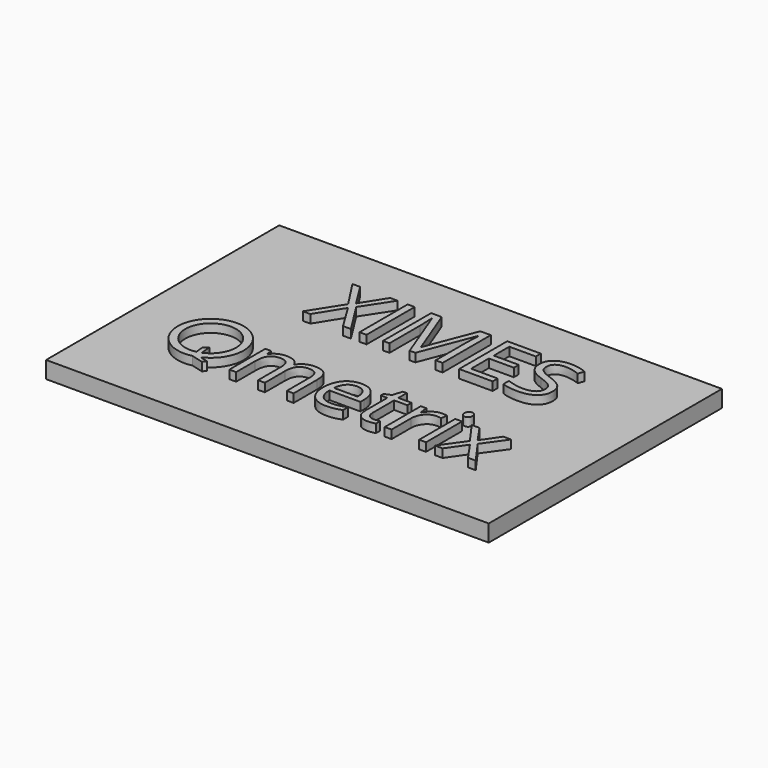
from build123d import *

# Parameters (mm, degrees)
F0_W         = 261.7531362921
F0_H         = 172.3503917456
F0_W_2       = 4.0420560748
F0_H_2       = 26.6744548287
F0_W_3       = 4.1355140187
F0_H_3       = 35.5841121495
F1_DEPTH     = 10
F0_TEXT_SIZE = 49.8442367601
F2_DEPTH     = 15


# Not quite as in the source:
# - Text() gives the source's letters only with a copy of the font that has no kerning and outlines rounded to 1/6400 em; it was checked with that copy


with BuildPart() as f1:
    # F0 (on Top) → F1 (new body)
    with BuildSketch(Plane.XY):
        with Locations((29.5447735116, 5.9954747558)):
            Rectangle(F0_W, F0_H)
        with BuildLine():
            ThreePointArc((-45.0583331062, -42.3228889704), (-55.8059475031, -4.8705779818), (-41.2665927015, -41.0201834508))
            Line((-41.2665927015, -41.0201834508), (-36.3650284708, -42.3228889704))
            Line((-36.3650284708, -42.3228889704), (-37.9992168005, -44.1990144973))
            Line((-37.9992168005, -44.1990144973), (-45.0583331062, -42.3228889704))
        make_face(mode=Mode.SUBTRACT)
        with BuildLine():
            Line((14.8038502761, -42.3830400759), (10.7695823634, -42.3830400759))
            Line((10.7695823634, -42.3830400759), (10.7695823634, -25.0310151538))
            add(Edge.make_bspline(
                [(10.7695823634, -25.0310151538), (10.7695823634, -21.8378687364), (9.4066540145, -20.2451896086)],
                knots=[0, 0, 0, 1, 1, 1], degree=2))
            add(Edge.make_bspline(
                [(9.4066540145, -20.2451896086), (8.0437256656, -18.6525104809), (5.1698938899, -18.6525104809)],
                knots=[0, 0, 0, 1, 1, 1], degree=2))
            add(Edge.make_bspline(
                [(5.1698938899, -18.6525104809), (1.4004234849, -18.6525104809), (-0.4025360167, -20.8176195152)],
                knots=[0, 0, 0, 1, 1, 1], degree=2))
            add(Edge.make_bspline(
                [(-0.4025360167, -20.8176195152), (-2.2054955182, -22.9827285495), (-2.2054955182, -27.4842861819)],
                knots=[0, 0, 0, 1, 1, 1], degree=2))
            Line((-2.2054955182, -27.4842861819), (-2.2054955182, -42.3830400759))
            Line((-2.2054955182, -42.3830400759), (-6.247551593, -42.3830400759))
            Line((-6.247551593, -42.3830400759), (-6.247551593, -25.0310151538))
            add(Edge.make_bspline(
                [(-6.247551593, -25.0310151538), (-6.247551593, -21.8378687364), (-7.6104799419, -20.2451896086)],
                knots=[0, 0, 0, 1, 1, 1], degree=2))
            add(Edge.make_bspline(
                [(-7.6104799419, -20.2451896086), (-8.9734082908, -18.6525104809), (-11.8706045525, -18.6525104809)],
                knots=[0, 0, 0, 1, 1, 1], degree=2))
            add(Edge.make_bspline(
                [(-11.8706045525, -18.6525104809), (-15.6634394435, -18.6525104809), (-17.4274581351, -20.9266537831)],
                knots=[0, 0, 0, 1, 1, 1], degree=2))
            add(Edge.make_bspline(
                [(-17.4274581351, -20.9266537831), (-19.1914768267, -23.2007970853), (-19.1914768267, -28.3877129731)],
                knots=[0, 0, 0, 1, 1, 1], degree=2))
            Line((-19.1914768267, -28.3877129731), (-19.1914768267, -42.3830400759))
            Line((-19.1914768267, -42.3830400759), (-23.2335329014, -42.3830400759))
            Line((-23.2335329014, -42.3830400759), (-23.2335329014, -15.7085852473))
            Line((-23.2335329014, -15.7085852473), (-19.9469285401, -15.7085852473))
            Line((-19.9469285401, -15.7085852473), (-19.2927229326, -19.3612332224))
            Line((-19.2927229326, -19.3612332224), (-19.0980188827, -19.3612332224))
            add(Edge.make_bspline(
                [(-19.0980188827, -19.3612332224), (-17.9531590696, -17.4141927239), (-15.8698257363, -16.3160618828)],
                knots=[0, 0, 0, 1, 1, 1], degree=2))
            add(Edge.make_bspline(
                [(-15.8698257363, -16.3160618828), (-13.786492403, -15.2179310417), (-11.208610783, -15.2179310417)],
                knots=[0, 0, 0, 1, 1, 1], degree=2))
            add(Edge.make_bspline(
                [(-11.208610783, -15.2179310417), (-4.954716702, -15.2179310417), (-3.0310406896, -19.750641322)],
                knots=[0, 0, 0, 1, 1, 1], degree=2))
            Line((-3.0310406896, -19.750641322), (-2.8363366397, -19.750641322))
            add(Edge.make_bspline(
                [(-2.8363366397, -19.750641322), (-1.6447478547, -17.6556257457), (0.6177132045, -16.4367783937)],
                knots=[0, 0, 0, 1, 1, 1], degree=2))
            add(Edge.make_bspline(
                [(0.6177132045, -16.4367783937), (2.8801742637, -15.2179310417), (5.7773705254, -15.2179310417)],
                knots=[0, 0, 0, 1, 1, 1], degree=2))
            add(Edge.make_bspline(
                [(5.7773705254, -15.2179310417), (10.3022926437, -15.2179310417), (12.5530714599, -17.5426973968)],
                knots=[0, 0, 0, 1, 1, 1], degree=2))
            add(Edge.make_bspline(
                [(12.5530714599, -17.5426973968), (14.8038502761, -19.8674637519), (14.8038502761, -24.9842861819)],
                knots=[0, 0, 0, 1, 1, 1], degree=2))
            Line((14.8038502761, -24.9842861819), (14.8038502761, -42.3830400759))
        make_face(mode=Mode.SUBTRACT)
        with BuildLine():
            add(Edge.make_bspline(
                [(39.0094577528, -42.4687098579), (37.1013580643, -42.8736942815), (34.3988658525, -42.8736942815)],
                knots=[0, 0, 0, 1, 1, 1], degree=2))
            add(Edge.make_bspline(
                [(34.3988658525, -42.8736942815), (28.4876508992, -42.8736942815), (25.0647537029, -39.2677752784)],
                knots=[0, 0, 0, 1, 1, 1], degree=2))
            add(Edge.make_bspline(
                [(25.0647537029, -39.2677752784), (21.6418565067, -35.6618562753), (21.6418565067, -29.2677752784)],
                knots=[0, 0, 0, 1, 1, 1], degree=2))
            add(Edge.make_bspline(
                [(21.6418565067, -29.2677752784), (21.6418565067, -22.8113889856), (24.8194266001, -19.0146600136)],
                knots=[0, 0, 0, 1, 1, 1], degree=2))
            add(Edge.make_bspline(
                [(24.8194266001, -19.0146600136), (27.9969966936, -15.2179310417), (33.3552521453, -15.2179310417)],
                knots=[0, 0, 0, 1, 1, 1], degree=2))
            add(Edge.make_bspline(
                [(33.3552521453, -15.2179310417), (38.3630403073, -15.2179310417), (41.283601055, -18.516217646)],
                knots=[0, 0, 0, 1, 1, 1], degree=2))
            add(Edge.make_bspline(
                [(41.283601055, -18.516217646), (44.2041618026, -21.8145042504), (44.2041618026, -27.2194886741)],
                knots=[0, 0, 0, 1, 1, 1], degree=2))
            Line((44.2041618026, -27.2194886741), (44.2041618026, -29.774005808))
            Line((44.2041618026, -29.774005808), (25.8318876593, -29.774005808))
            add(Edge.make_bspline(
                [(25.8318876593, -29.774005808), (25.9564982512, -34.4702674903), (28.2072770674, -36.9040681133)],
                knots=[0, 0, 0, 1, 1, 1], degree=2))
            add(Edge.make_bspline(
                [(28.2072770674, -36.9040681133), (30.4580558836, -39.3378687364), (34.5468409304, -39.3378687364)],
                knots=[0, 0, 0, 1, 1, 1], degree=2))
            add(Edge.make_bspline(
                [(34.5468409304, -39.3378687364), (38.8536945129, -39.3378687364), (43.0593019895, -37.5388033158)],
                knots=[0, 0, 0, 1, 1, 1], degree=2))
            Line((43.0593019895, -37.5388033158), (43.0593019895, -41.1447223189))
            add(Edge.make_bspline(
                [(43.0593019895, -41.1447223189), (40.9175574413, -42.0637254342), (39.0094577528, -42.4687098579)],
                knots=[0, 0, 0, 1, 1, 1], degree=2))
        make_face(mode=Mode.SUBTRACT)
        with BuildLine():
            add(Edge.make_bspline(
                [(56.5717630487, -38.2436319762), (57.7166228618, -39.5325727862), (59.7103923322, -39.5325727862)],
                knots=[0, 0, 0, 1, 1, 1], degree=2))
            add(Edge.make_bspline(
                [(59.7103923322, -39.5325727862), (60.7851586874, -39.5325727862), (61.7820434226, -39.3768095463)],
                knots=[0, 0, 0, 1, 1, 1], degree=2))
            add(Edge.make_bspline(
                [(61.7820434226, -39.3768095463), (62.7789281578, -39.2210463065), (63.3630403073, -39.0497067426)],
                knots=[0, 0, 0, 1, 1, 1], degree=2))
            Line((63.3630403073, -39.0497067426), (63.3630403073, -42.1416070541))
            add(Edge.make_bspline(
                [(63.3630403073, -42.1416070541), (62.7088346998, -42.4531335339), (61.4315761328, -42.6634139077)],
                knots=[0, 0, 0, 1, 1, 1], degree=2))
            add(Edge.make_bspline(
                [(61.4315761328, -42.6634139077), (60.1543175659, -42.8736942815), (59.1262801827, -42.8736942815)],
                knots=[0, 0, 0, 1, 1, 1], degree=2))
            add(Edge.make_bspline(
                [(59.1262801827, -42.8736942815), (51.3926353229, -42.8736942815), (51.3926353229, -34.7194886741)],
                knots=[0, 0, 0, 1, 1, 1], degree=2))
            Line((51.3926353229, -34.7194886741), (51.3926353229, -18.8472145308))
            Line((51.3926353229, -18.8472145308), (47.5686477839, -18.8472145308))
            Line((47.5686477839, -18.8472145308), (47.5686477839, -16.9001740323))
            Line((47.5686477839, -16.9001740323), (51.3926353229, -15.2179310417))
            Line((51.3926353229, -15.2179310417), (53.0904546375, -9.5247846242))
            Line((53.0904546375, -9.5247846242), (55.4269032356, -9.5247846242))
            Line((55.4269032356, -9.5247846242), (55.4269032356, -15.7085852473))
            Line((55.4269032356, -15.7085852473), (63.1683362575, -15.7085852473))
            Line((63.1683362575, -15.7085852473), (63.1683362575, -18.8472145308))
            Line((63.1683362575, -18.8472145308), (55.4269032356, -18.8472145308))
            Line((55.4269032356, -18.8472145308), (55.4269032356, -34.5481491102))
            add(Edge.make_bspline(
                [(55.4269032356, -34.5481491102), (55.4269032356, -36.9546911663), (56.5717630487, -38.2436319762)],
                knots=[0, 0, 0, 1, 1, 1], degree=2))
        make_face(mode=Mode.SUBTRACT)
        with BuildLine():
            add(Edge.make_bspline(
                [(76.260236569, -16.6314824435), (78.3552521453, -15.2179310417), (80.8630403073, -15.2179310417)],
                knots=[0, 0, 0, 1, 1, 1], degree=2))
            add(Edge.make_bspline(
                [(80.8630403073, -15.2179310417), (82.6387412419, -15.2179310417), (84.0483985628, -15.5138811974)],
                knots=[0, 0, 0, 1, 1, 1], degree=2))
            Line((84.0483985628, -15.5138811974), (83.4876508992, -19.2599871164))
            add(Edge.make_bspline(
                [(83.4876508992, -19.2599871164), (81.8365605565, -18.8939435027), (80.5670901515, -18.8939435027)],
                knots=[0, 0, 0, 1, 1, 1], degree=2))
            add(Edge.make_bspline(
                [(80.5670901515, -18.8939435027), (77.3272147621, -18.8939435027), (75.029706974, -21.5224481756)],
                knots=[0, 0, 0, 1, 1, 1], degree=2))
            add(Edge.make_bspline(
                [(75.029706974, -21.5224481756), (72.7321991858, -24.1509528485), (72.7321991858, -28.0683983314)],
                knots=[0, 0, 0, 1, 1, 1], degree=2))
            Line((72.7321991858, -28.0683983314), (72.7321991858, -42.3830400759))
            Line((72.7321991858, -42.3830400759), (68.690143111, -42.3830400759))
            Line((68.690143111, -42.3830400759), (68.690143111, -15.7085852473))
            Line((68.690143111, -15.7085852473), (72.0234764444, -15.7085852473))
            Line((72.0234764444, -15.7085852473), (72.490766164, -20.6462799513))
            Line((72.490766164, -20.6462799513), (72.6854702138, -20.6462799513))
            add(Edge.make_bspline(
                [(72.6854702138, -20.6462799513), (74.1652209927, -18.0450338454), (76.260236569, -16.6314824435)],
                knots=[0, 0, 0, 1, 1, 1], degree=2))
        make_face(mode=Mode.SUBTRACT)
        with Locations((91.0616384381, -29.0458126616)):
            Rectangle(F0_W_2, F0_H_2, mode=Mode.SUBTRACT)
        with BuildLine():
            add(Edge.make_bspline(
                [(89.3793954475, -10.5138811974), (88.697931273, -9.844099266), (88.697931273, -8.4811709171)],
                knots=[0, 0, 0, 1, 1, 1], degree=2))
            add(Edge.make_bspline(
                [(88.697931273, -8.4811709171), (88.697931273, -7.0948780822), (89.3793954475, -6.4484606367)],
                knots=[0, 0, 0, 1, 1, 1], degree=2))
            add(Edge.make_bspline(
                [(89.3793954475, -6.4484606367), (90.0608596219, -5.8020431912), (91.0888970051, -5.8020431912)],
                knots=[0, 0, 0, 1, 1, 1], degree=2))
            add(Edge.make_bspline(
                [(91.0888970051, -5.8020431912), (92.0624172543, -5.8020431912), (92.7672459148, -6.4601428797)],
                knots=[0, 0, 0, 1, 1, 1], degree=2))
            add(Edge.make_bspline(
                [(92.7672459148, -6.4601428797), (93.4720745752, -7.1182425681), (93.4720745752, -8.4811709171)],
                knots=[0, 0, 0, 1, 1, 1], degree=2))
            add(Edge.make_bspline(
                [(93.4720745752, -8.4811709171), (93.4720745752, -9.844099266), (92.7672459148, -10.5138811974)],
                knots=[0, 0, 0, 1, 1, 1], degree=2))
            add(Edge.make_bspline(
                [(92.7672459148, -10.5138811974), (92.0624172543, -11.1836631289), (91.0888970051, -11.1836631289)],
                knots=[0, 0, 0, 1, 1, 1], degree=2))
            add(Edge.make_bspline(
                [(91.0888970051, -11.1836631289), (90.0608596219, -11.1836631289), (89.3793954475, -10.5138811974)],
                knots=[0, 0, 0, 1, 1, 1], degree=2))
        make_face(mode=Mode.SUBTRACT)
        Polygon((98.3163113353, -42.3830400759), (108.0748783135, -28.7303921009), (98.799177379, -15.7085852473), (103.4019811173, -15.7085852473), (110.4346913976, -25.9266537831), (117.444037192, -15.7085852473), (122.0001119584, -15.7085852473), (112.7244110238, -28.7303921009), (122.482978002, -42.3830400759), (117.9113269117, -42.3830400759), (110.4346913976, -31.5730712286), (102.8879624257, -42.3830400759), align=None, mode=Mode.SUBTRACT)
        Polygon((-16.6011314449, 43.1183571619), (-4.7241844044, 24.3800394049), (-9.4204460866, 24.3800394049), (-18.984309015, 40.0264568504), (-28.7195115072, 24.3800394049), (-33.1042467097, 24.3800394049), (-21.2740286411, 42.978170246), (-32.3020660243, 59.9641515544), (-27.722626772, 59.9641515544), (-18.8908510711, 45.8675783457), (-9.9811937502, 59.9641515544), (-5.5808822237, 59.9641515544), align=None, mode=Mode.SUBTRACT)
        with Locations((2.4292423869, 42.1720954797)):
            Rectangle(F0_W_3, F0_H_3, mode=Mode.SUBTRACT)
        with BuildLine():
            Line((33.3365632592, 24.3800394049), (30.0032299258, 24.3800394049))
            Line((30.0032299258, 24.3800394049), (17.9315788355, 55.9220954797))
            Line((17.9315788355, 55.9220954797), (17.7368747856, 55.9220954797))
            add(Edge.make_bspline(
                [(17.7368747856, 55.9220954797), (18.0795539134, 52.1759895607), (18.0795539134, 47.0124381588)],
                knots=[0, 0, 0, 1, 1, 1], degree=2))
            Line((18.0795539134, 47.0124381588), (18.0795539134, 24.3800394049))
            Line((18.0795539134, 24.3800394049), (14.2555663744, 24.3800394049))
            Line((14.2555663744, 24.3800394049), (14.2555663744, 59.9641515544))
            Line((14.2555663744, 59.9641515544), (20.4860959694, 59.9641515544))
            Line((20.4860959694, 59.9641515544), (31.7555663744, 30.6105689999))
            Line((31.7555663744, 30.6105689999), (31.9502704243, 30.6105689999))
            Line((31.9502704243, 30.6105689999), (43.3131987732, 59.9641515544))
            Line((43.3131987732, 59.9641515544), (49.4969993962, 59.9641515544))
            Line((49.4969993962, 59.9641515544), (49.4969993962, 24.3800394049))
            Line((49.4969993962, 24.3800394049), (45.3614853775, 24.3800394049))
            Line((45.3614853775, 24.3800394049), (45.3614853775, 47.3083883146))
            add(Edge.make_bspline(
                [(45.3614853775, 47.3083883146), (45.3614853775, 51.2491982834), (45.7041645053, 55.8753665077)],
                knots=[0, 0, 0, 1, 1, 1], degree=2))
            Line((45.7041645053, 55.8753665077), (45.5094604554, 55.8753665077))
            Line((45.5094604554, 55.8753665077), (33.3365632592, 24.3800394049))
        make_face(mode=Mode.SUBTRACT)
        Polygon((79.0920149726, 28.0794163519), (79.0920149726, 24.3800394049), (59.2555663744, 24.3800394049), (59.2555663744, 59.9641515544), (79.0920149726, 59.9641515544), (79.0920149726, 56.2881390934), (63.3910803931, 56.2881390934), (63.3910803931, 44.8239646385), (78.1418592093, 44.8239646385), (78.1418592093, 41.1713166635), (63.3910803931, 41.1713166635), (63.3910803931, 28.0794163519), align=None, mode=Mode.SUBTRACT)
        with BuildLine():
            add(Edge.make_bspline(
                [(104.9487127919, 39.7850238286), (107.0515165302, 37.4953042024), (107.0515165302, 33.8504443893)],
                knots=[0, 0, 0, 1, 1, 1], degree=2))
            add(Edge.make_bspline(
                [(107.0515165302, 33.8504443893), (107.0515165302, 29.1541827071), (103.6441956579, 26.5217839532)],
                knots=[0, 0, 0, 1, 1, 1], degree=2))
            add(Edge.make_bspline(
                [(103.6441956579, 26.5217839532), (100.2368747856, 23.8893851993), (94.3957532903, 23.8893851993)],
                knots=[0, 0, 0, 1, 1, 1], degree=2))
            add(Edge.make_bspline(
                [(94.3957532903, 23.8893851993), (88.0717657514, 23.8893851993), (84.6605507981, 25.524899218)],
                knots=[0, 0, 0, 1, 1, 1], degree=2))
            Line((84.6605507981, 25.524899218), (84.6605507981, 29.5124381588))
            add(Edge.make_bspline(
                [(84.6605507981, 29.5124381588), (86.8568124803, 28.5934350435), (89.4346941003, 28.056051866)],
                knots=[0, 0, 0, 1, 1, 1], degree=2))
            add(Edge.make_bspline(
                [(89.4346941003, 28.056051866), (92.0125757202, 27.5186686884), (94.5437283682, 27.5186686884)],
                knots=[0, 0, 0, 1, 1, 1], degree=2))
            add(Edge.make_bspline(
                [(94.5437283682, 27.5186686884), (98.6792423869, 27.5186686884), (100.7742579632, 29.0879833301)],
                knots=[0, 0, 0, 1, 1, 1], degree=2))
            add(Edge.make_bspline(
                [(100.7742579632, 29.0879833301), (102.8692735395, 30.6572979719), (102.8692735395, 33.4610362896)],
                knots=[0, 0, 0, 1, 1, 1], degree=2))
            add(Edge.make_bspline(
                [(102.8692735395, 33.4610362896), (102.8692735395, 35.3068306822), (102.1255040691, 36.4867372242)],
                knots=[0, 0, 0, 1, 1, 1], degree=2))
            add(Edge.make_bspline(
                [(102.1255040691, 36.4867372242), (101.3817345987, 37.6666437663), (99.6410803931, 38.6674225825)],
                knots=[0, 0, 0, 1, 1, 1], degree=2))
            add(Edge.make_bspline(
                [(99.6410803931, 38.6674225825), (97.9004261875, 39.6682013987), (94.3490243184, 40.9298836417)],
                knots=[0, 0, 0, 1, 1, 1], degree=2))
            add(Edge.make_bspline(
                [(94.3490243184, 40.9298836417), (89.3879651283, 42.7055845762), (87.257902823, 45.1393851993)],
                knots=[0, 0, 0, 1, 1, 1], degree=2))
            add(Edge.make_bspline(
                [(87.257902823, 45.1393851993), (85.1278405177, 47.5731858223), (85.1278405177, 51.4906313052)],
                knots=[0, 0, 0, 1, 1, 1], degree=2))
            add(Edge.make_bspline(
                [(85.1278405177, 51.4906313052), (85.1278405177, 55.6027808379), (88.2158467483, 58.036581461)],
                knots=[0, 0, 0, 1, 1, 1], degree=2))
            add(Edge.make_bspline(
                [(88.2158467483, 58.036581461), (91.3038529788, 60.470382084), (96.3973109227, 60.470382084)],
                knots=[0, 0, 0, 1, 1, 1], degree=2))
            add(Edge.make_bspline(
                [(96.3973109227, 60.470382084), (101.7010492405, 60.470382084), (106.1558779009, 58.5233415856)],
                knots=[0, 0, 0, 1, 1, 1], degree=2))
            Line((106.1558779009, 58.5233415856), (104.8630430099, 54.9252107445))
            add(Edge.make_bspline(
                [(104.8630430099, 54.9252107445), (100.4549433215, 56.771005137), (96.2960648168, 56.771005137)],
                knots=[0, 0, 0, 1, 1, 1], degree=2))
            add(Edge.make_bspline(
                [(96.2960648168, 56.771005137), (93.0094604554, 56.771005137), (91.1597719819, 55.3613478161)],
                knots=[0, 0, 0, 1, 1, 1], degree=2))
            add(Edge.make_bspline(
                [(91.1597719819, 55.3613478161), (89.3100835084, 53.9516904952), (89.3100835084, 51.4439023333)],
                knots=[0, 0, 0, 1, 1, 1], degree=2))
            add(Edge.make_bspline(
                [(89.3100835084, 51.4439023333), (89.3100835084, 49.5981079407), (89.9915476828, 48.4143073177)],
                knots=[0, 0, 0, 1, 1, 1], degree=2))
            add(Edge.make_bspline(
                [(89.9915476828, 48.4143073177), (90.6730118573, 47.2305066946), (92.292949552, 46.2453042024)],
                knots=[0, 0, 0, 1, 1, 1], degree=2))
            add(Edge.make_bspline(
                [(92.292949552, 46.2453042024), (93.9128872467, 45.2601017102), (97.24622058, 44.0685129252)],
                knots=[0, 0, 0, 1, 1, 1], degree=2))
            add(Edge.make_bspline(
                [(97.24622058, 44.0685129252), (102.8459090536, 42.0747434547), (104.9487127919, 39.7850238286)],
                knots=[0, 0, 0, 1, 1, 1], degree=2))
        make_face(mode=Mode.SUBTRACT)
    extrude(amount=F1_DEPTH)



with BuildPart() as f1b:
    # F0 (on Top) → F1, piece 2 (new body)
    with BuildSketch(Plane.XY):
        with BuildLine():
            ThreePointArc((-43.7490858011, -37.1871398378), (-53.9394303244, -9.0020291393), (-46.276672768, -37.9765995973))
            Line((-46.276672768, -37.9765995973), (-46.6589570613, -33.0732026998))
            Line((-46.6589570613, -33.0732026998), (-44.2494047513, -30.769762951))
            Line((-44.2494047513, -30.769762951), (-43.7490858011, -37.1871398378))
        make_face()
    extrude(amount=F1_DEPTH)


with BuildPart() as f1c:
    # F0 (on Top) → F1, piece 3 (new body)
    with BuildSketch(Plane.XY):
        with BuildLine():
            add(Edge.make_bspline(
                [(38.1722303385, -20.6384917893), (36.4705169428, -18.605781509), (33.3007350114, -18.605781509)],
                knots=[0, 0, 0, 1, 1, 1], degree=2))
            add(Edge.make_bspline(
                [(33.3007350114, -18.605781509), (30.0920122699, -18.605781509), (28.1800185004, -20.6969030043)],
                knots=[0, 0, 0, 1, 1, 1], degree=2))
            add(Edge.make_bspline(
                [(28.1800185004, -20.6969030043), (26.268024731, -22.7880244996), (25.9253456033, -26.4874014467)],
                knots=[0, 0, 0, 1, 1, 1], degree=2))
            Line((25.9253456033, -26.4874014467), (39.8739437341, -26.4874014467))
            add(Edge.make_bspline(
                [(39.8739437341, -26.4874014467), (39.8739437341, -22.6712020697), (38.1722303385, -20.6384917893)],
                knots=[0, 0, 0, 1, 1, 1], degree=2))
        make_face()
    extrude(amount=F1_DEPTH)


with BuildPart() as f1_1:
    add(f1.part)

    add(f1b.part)  # F2 merges F1b

    add(f1c.part)  # F2 merges F1c
    # F0 (on Top) → F2 (join)
    with BuildSketch(Plane.XY):
        with BuildLine():
            Line((-36.3650284708, -42.3228889704), (-41.2665927015, -41.0201834508))
            ThreePointArc((-41.2665927015, -41.0201834508), (-55.8059475031, -4.8705779818), (-45.0583331062, -42.3228889704))
            Line((-45.0583331062, -42.3228889704), (-37.9992168005, -44.1990144973))
            Line((-37.9992168005, -44.1990144973), (-36.3650284708, -42.3228889704))
        make_face()
        with BuildLine():
            Line((-46.6589570613, -33.0732026998), (-46.276672768, -37.9765995973))
            ThreePointArc((-46.276672768, -37.9765995973), (-53.9394303244, -9.0020291393), (-43.7490858011, -37.1871398378))
            Line((-43.7490858011, -37.1871398378), (-44.2494047513, -30.769762951))
            Line((-44.2494047513, -30.769762951), (-46.6589570613, -33.0732026998))
        make_face(mode=Mode.SUBTRACT)
        with Locations((-27.517021998, -42.3830400759)):
            Text('metrix', F0_TEXT_SIZE, font='Open Sans', text_align=(TextAlign.LEFT, TextAlign.BOTTOM))
        with Locations((-33.2989507595, 24.3800394049)):
            Text('XIMES', F0_TEXT_SIZE, font='Open Sans', text_align=(TextAlign.LEFT, TextAlign.BOTTOM))
    extrude(amount=F2_DEPTH)


solid = f1_1.part
